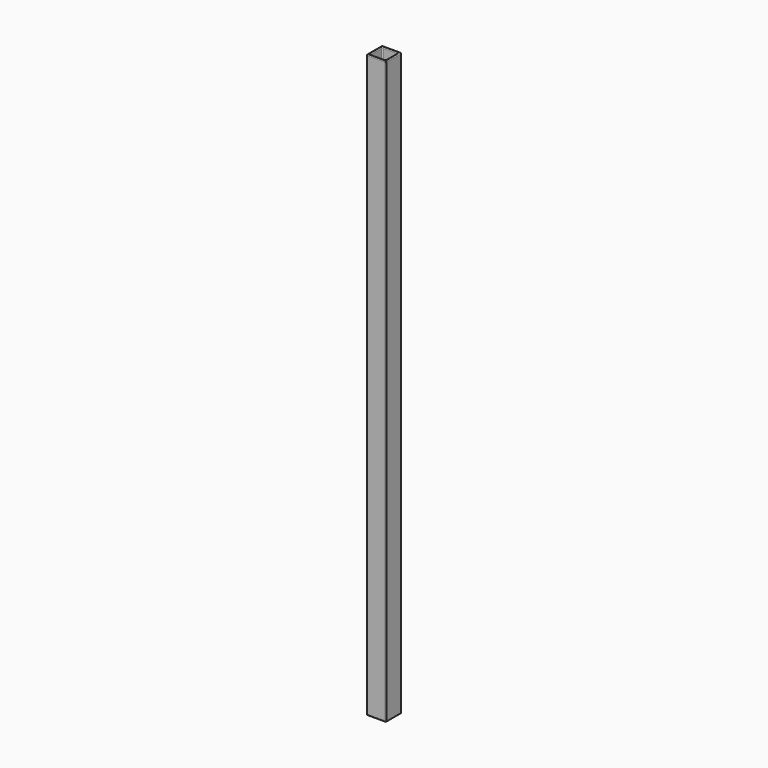
from build123d import *

# Parameters (mm, degrees)
F0_W         = 25.4
F0_H         = 25.4
F0_W_2       = 20.32
F0_H_2       = 20.32
F1_DEPTH     = 381
F2_R         = 1.26999
F3_T1_DEPTH  = 30.48001
F3_T3_DEPTH  = 768.35
F4_T1_DEPTH  = 26.03501
F4_T3_DEPTH  = 759.46
F4_T5_DEPTH  = 26.035
F4_S9_W      = 1.2954
F4_S9_H      = 1.2954
F4_T10_DEPTH = 1.2954
F4_S15_W     = 1.2954
F4_S15_H     = 1.2954
F4_T16_DEPTH = 1.2954


# Not quite as in the source:
# - a fillet or chamfer that OpenCascade refuses, or shapes differently, is made with other operations: its cross-section is extruded or revolved along the edge and cut away or added
# - a fillet or chamfer is up to 0.001 mm smaller than in the source, because OpenCascade refuses the exact size


with BuildPart() as f1:
    # F0 (on Top) → F1 (new body, symmetric)
    with BuildSketch(Plane.XY):
        Rectangle(F0_W, F0_H)
        Rectangle(F0_W_2, F0_H_2, mode=Mode.SUBTRACT)
    extrude(amount=F1_DEPTH, both=True)

    # F2 (radius 1.27 in the source; OpenCascade refuses exactly that, so slightly less here)
    f2_edges = [f1.edges().sort_by_distance(p)[0] for p in [
        (0, -10.16, -381),
        (-10.16, -10.16, 0),
        (0, -10.16, 381),
        (10.16, -10.16, 0),
        (10.16, 10.16, 0),
        (10.16, 0, -381),
        (10.16, 0, 381),
        (-10.16, 0, -381),
        (-10.16, 10.16, 0),
        (-10.16, 0, 381),
        (0, 10.16, -381),
        (0, 10.16, 381),
        (12.7, -12.7, 0),
        (12.7, 0, -381),
        (12.7, 12.7, 0),
        (12.7, 0, 381),
    ]]
    fillet(f2_edges, radius=F2_R)

    # F3: fillet of radius 1.27 on 8 edges, made by hand

    # F3_s2 → F3_t1 (cut)
    with BuildSketch(Plane.YZ.offset(-15.875)):
        with BuildLine():
            ThreePointArc((-11.43, -381), (-12.3280256121, -380.6280256121), (-12.7, -379.73))
            Line((-12.7, -379.73), (-12.7, -381))
            Line((-12.7, -381), (-11.43, -381))
        make_face()
        with BuildLine():
            ThreePointArc((-11.43, 381), (-12.3280256121, 380.6280256121), (-12.7, 379.73))
            Line((-12.7, 379.73), (-12.7, 381))
            Line((-12.7, 381), (-11.43, 381))
        make_face()
    extrude(amount=F3_T1_DEPTH, mode=Mode.SUBTRACT)

    # F3_s4 → F3_t3 (cut)
    with BuildSketch(Plane.XY.offset(-384.175)):
        with BuildLine():
            ThreePointArc((-12.7, -11.43), (-12.3280256121, -12.3280256121), (-11.43, -12.7))
            Line((-11.43, -12.7), (-12.7, -12.7))
            Line((-12.7, -12.7), (-12.7, -11.43))
        make_face()
    extrude(amount=F3_T3_DEPTH, mode=Mode.SUBTRACT)

    # F4: fillet of radius 1.27 on 7 edges, made by hand

    # F4_s2 → F4_t1 (cut)
    with BuildSketch(Plane.YZ.offset(-11.43)):
        with BuildLine():
            ThreePointArc((12.7, -379.73), (12.3280256121, -380.6280256121), (11.43, -381))
            Line((11.43, -381), (12.7, -381))
            Line((12.7, -381), (12.7, -379.73))
        make_face()
        with BuildLine():
            ThreePointArc((12.7, 379.73), (12.3280256121, 380.6280256121), (11.43, 381))
            Line((11.43, 381), (12.7, 381))
            Line((12.7, 381), (12.7, 379.73))
        make_face()
    extrude(amount=F4_T1_DEPTH, mode=Mode.SUBTRACT)

    # F4_s4 → F4_t3 (cut)
    with BuildSketch(Plane.XY.offset(-379.73)):
        with BuildLine():
            ThreePointArc((-11.43, 12.7), (-12.3280256121, 12.3280256121), (-12.7, 11.43))
            Line((-12.7, 11.43), (-12.7, 12.7))
            Line((-12.7, 12.7), (-11.43, 12.7))
        make_face()
    extrude(amount=F4_T3_DEPTH, mode=Mode.SUBTRACT)

    # F4_s6 → F4_t5 (cut)
    with BuildSketch(Plane.XZ.offset(-11.43)):
        with BuildLine():
            ThreePointArc((-12.7, 379.73), (-12.3280256121, 380.6280256121), (-11.43, 381))
            Line((-11.43, 381), (-12.7, 381))
            Line((-12.7, 381), (-12.7, 379.73))
        make_face()
        with BuildLine():
            ThreePointArc((-11.43, -381), (-12.3280256121, -380.6280256121), (-12.7, -379.73))
            Line((-12.7, -379.73), (-12.7, -381))
            Line((-12.7, -381), (-11.43, -381))
        make_face()
    extrude(amount=F4_T5_DEPTH, mode=Mode.SUBTRACT)


with BuildPart() as f4_tool8:
    # F4_s9 → F4_t10 (new body)
    with BuildSketch(Plane.XZ.offset(-11.43)):
        with Locations((-12.0777, -380.3777)):
            Rectangle(F4_S9_W, F4_S9_H)
    extrude(amount=-F4_T10_DEPTH)

    # F4_s11 → F4_t12 (revolve, cut)
    with BuildSketch(Plane(origin=(-11.43, 11.43, -379.73), x_dir=(0.7071067812, 0, 0.7071067812), z_dir=(-0.7071067812, 0, 0.7071067812))):
        with BuildLine():
            ThreePointArc((0, -1.27), (1.27, 0), (0, 1.27))
            Line((0, 1.27), (0, -1.27))
        make_face()
    revolve(axis=Axis((-11.43, 11.43, -379.73), (0, 1, 0)), mode=Mode.SUBTRACT)


with BuildPart() as f1_1:
    add(f1.part)

    # F4_t7: cut F4_tool8
    add(f4_tool8.part, mode=Mode.SUBTRACT)


with BuildPart() as f4_tool14:
    # F4_s15 → F4_t16 (new body)
    with BuildSketch(Plane.XZ.offset(-11.43)):
        with Locations((-12.0777, 380.3777)):
            Rectangle(F4_S15_W, F4_S15_H)
    extrude(amount=-F4_T16_DEPTH)

    # F4_s17 → F4_t18 (revolve, cut)
    with BuildSketch(Plane(origin=(-11.43, 11.43, 379.73), x_dir=(0.7071067812, 0, -0.7071067812), z_dir=(0.7071067812, 0, 0.7071067812))):
        with BuildLine():
            ThreePointArc((0, -1.27), (1.27, 0), (0, 1.27))
            Line((0, 1.27), (0, -1.27))
        make_face()
    revolve(axis=Axis((-11.43, 11.43, 379.73), (0, 1, 0)), mode=Mode.SUBTRACT)


with BuildPart() as f1_2:
    add(f1_1.part)

    # F4_t13: cut F4_tool14
    add(f4_tool14.part, mode=Mode.SUBTRACT)


solid = f1_2.part
